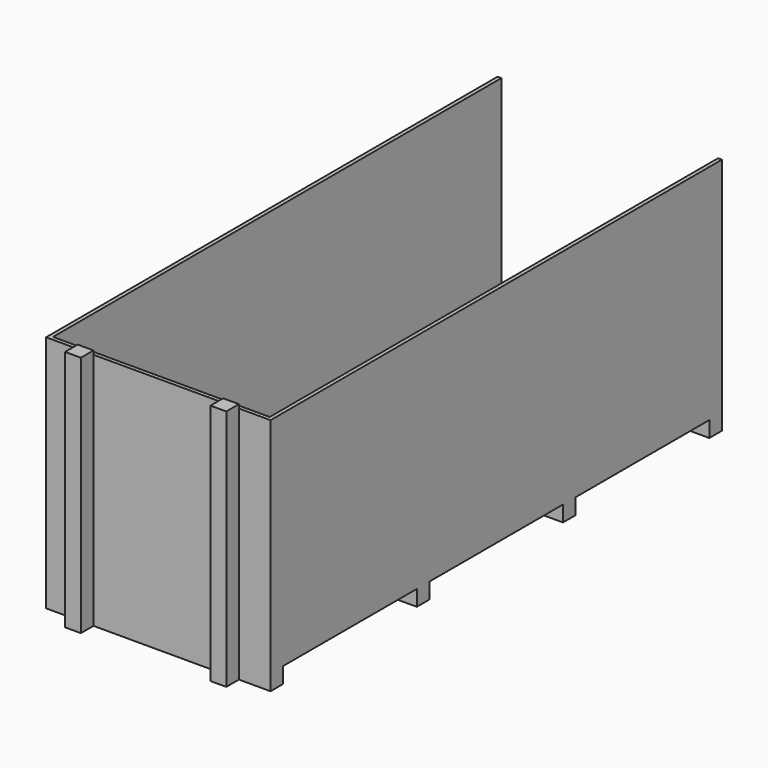
from build123d import *

# Parameters (mm, degrees)
F0_W     = 994
F0_H     = 2499
F1_DEPTH = 987
F2_W     = 960
F2_H     = 2482
F3_DEPTH = 970
F5_W     = 70
F5_H     = 70
F6_DEPTH = 1074
F7_W     = 994
F7_H     = 70
F8_DEPTH = 70


with BuildPart() as f1:
    # F0 (on Top) → F1 (new body)
    with BuildSketch(Plane.XY):
        Rectangle(F0_W, F0_H)
    extrude(amount=-F1_DEPTH)

    # F2 (on Top) → F3 (cut)
    with BuildSketch(Plane.XY):
        with Locations((0, 8.5)):
            Rectangle(F2_W, F2_H)
    extrude(amount=-F3_DEPTH, mode=Mode.SUBTRACT)

    # F7 (on face) → F8 (join)
    with BuildSketch(Plane(origin=(0, 0, -987), x_dir=(1, 0, 0), z_dir=(0, 0, -1))):
        with Locations((0, -1214.5)):
            Rectangle(F7_W, F7_H)
        with Locations((0, -404.5)):
            Rectangle(F7_W, F7_H)
        with Locations((0, 1214.5)):
            Rectangle(F7_W, F7_H)
        with Locations((0, 404.5)):
            Rectangle(F7_W, F7_H)
    extrude(amount=F8_DEPTH)


with BuildPart() as f6:
    # F5 (on offset) → F6 (new body)
    with BuildSketch(Plane.XY.offset(17)):
        with Locations((-322, -1284.5)):
            Rectangle(F5_W, F5_H)
    extrude(amount=-F6_DEPTH)


with BuildPart() as f6b:
    # F5 (on offset) → F6, piece 2 (new body)
    with BuildSketch(Plane.XY.offset(17)):
        with Locations((322, -1284.5)):
            Rectangle(F5_W, F5_H)
    extrude(amount=-F6_DEPTH)


solid = Compound([f1.part, f6.part, f6b.part])
